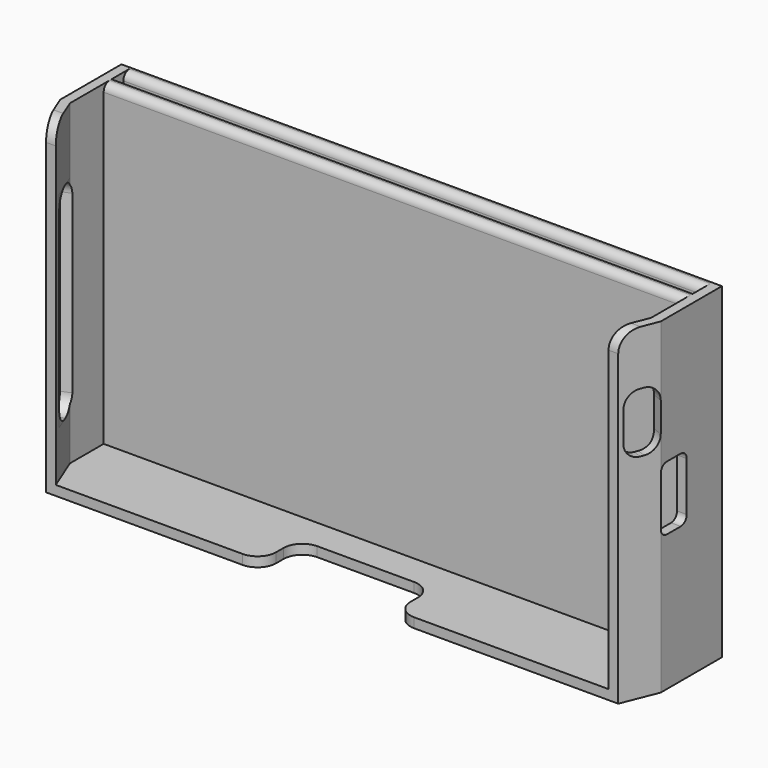
from build123d import *

# Parameters (mm, degrees)
F0_W          = 155.8
F0_H          = 85
F1_DEPTH      = 2.6
F3_DEPTH      = 85
F5_DEPTH      = 2.6
F6_W          = 8.7
F6_H          = 17.2
F7_DEPTH      = 25
F8_W          = 9
F8_H          = 16
F9_DEPTH      = 25
F10_W         = 8.5
F10_H         = 55.1
F11_DEPTH     = 25
F12_W         = 6.6
F12_H         = 87.6
F13_DEPTH     = 2.6
F14_W         = 6.6
F14_H         = 87.6
F15_DEPTH     = 2.6
F16_W         = 155.8
F16_H         = 87.6
F17_DEPTH     = 2.6
F19_W         = 36
F19_H         = 12.5
F20_DEPTH     = 25
F21_T1_DEPTH  = 2.4140393963
F21_T6_DEPTH  = 12.7075604463
F21_T12_DEPTH = 12.7075604463
F21_T18_DEPTH = 12.7075604463
F21_T24_DEPTH = 12.7075604463
F21_T30_DEPTH = 12.7075604463
F21_T36_DEPTH = 12.7075604463
F22_R         = 4
F23_T1_DEPTH  = 2.6
F23_T6_DEPTH  = 2.6
F23_T12_DEPTH = 2.6
F23_T17_DEPTH = 2.6
F23_T23_DEPTH = 2.6
F24_R         = 5
F25_R         = 2
F26_R         = 5


# Not quite as in the source:
# - a fillet or chamfer that OpenCascade refuses, or shapes differently, is made with other operations: its cross-section is extruded or revolved along the edge and cut away or added


with BuildPart() as f1:
    # F0 (on Front) → F1 (new body)
    with BuildSketch(Plane.XZ):
        Rectangle(F0_W, F0_H)
    extrude(amount=F1_DEPTH)

    # F2 (on face) → F3 (join)
    with BuildSketch(Plane.XY.offset(42.5)):
        Polygon((-77.9, -13.9), (-77.9, -2.6), (-77.9, 0), (-80.5, 0), (-80.5, -13.9), align=None)
        Polygon((-74.1, -23.4), (-77.9, -13.9), (-80.5, -13.9), (-76.7, -23.4), align=None)
        Polygon((77.9, 0), (77.9, -2.6), (77.9, -13.9), (74.1, -23.4), (76.7, -23.4), (80.5, -13.9), (80.5, 0), align=None)
    extrude(amount=-F3_DEPTH)

    # F4 (on face) → F5 (join)
    with BuildSketch(Plane(origin=(0, 0, -42.5), x_dir=(1, 0, 0), z_dir=(0, 0, -1))):
        Polygon((74.1, 23.4), (-74.1, 23.4), (-77.9, 13.9), (-77.9, 2.6), (77.9, 2.6), (77.9, 13.9), align=None)
        Polygon((-77.9, 13.9), (-74.1, 23.4), (-76.7, 23.4), (-80.5, 13.9), (-80.5, 0), (80.5, 0), (80.5, 13.9), (76.7, 23.4), (74.1, 23.4), (77.9, 13.9), (77.9, 2.6), (-77.9, 2.6), align=None)
    extrude(amount=F5_DEPTH)

    # F6 (on face) → F7 (cut)
    with BuildSketch(Plane.YZ.offset(80.5)):
        with Locations((-9.55, 0)):
            Rectangle(F6_W, F6_H)
    extrude(amount=-F7_DEPTH, mode=Mode.SUBTRACT)

    # F8 (on face) → F9 (cut)
    with BuildSketch(Plane(origin=(74.1896551724, -29.675862069, 0), x_dir=(0.3713906764, 0.9284766909, 0), z_dir=(0.9284766909, -0.3713906764, 0))):
        with Locations((12.4911234432, 19.9)):
            Rectangle(F8_W, F8_H)
    extrude(amount=-F9_DEPTH, mode=Mode.SUBTRACT)

    # F10 (on face) → F11 (cut)
    with BuildSketch(Plane(origin=(-74.1896551724, -29.675862069, 0), x_dir=(0.3713906764, -0.9284766909, 0), z_dir=(-0.9284766909, -0.3713906764, 0))):
        with Locations((-12.5093103096, -2.65)):
            Rectangle(F10_W, F10_H)
    extrude(amount=-F11_DEPTH, mode=Mode.SUBTRACT)

    # F12 (on face) → F13 (join)
    with BuildSketch(Plane(origin=(-80.5, 0, 0), x_dir=(0, -1, 0), z_dir=(-1, 0, 0))):
        with Locations((-3.3, -1.3)):
            Rectangle(F12_W, F12_H)
    extrude(amount=-F13_DEPTH)

    # F14 (on face) → F15 (join)
    with BuildSketch(Plane.YZ.offset(80.5)):
        with Locations((3.3, -1.3)):
            Rectangle(F14_W, F14_H)
    extrude(amount=-F15_DEPTH)

    # F16 (on face) → F17 (join)
    with BuildSketch(Plane(origin=(0, 6.6, 0), x_dir=(-1, 0, 0), z_dir=(0, 1, 0))):
        with Locations((0, -1.3)):
            Rectangle(F16_W, F16_H)
    extrude(amount=-F17_DEPTH)

    # F18: union 

    # F19 (on face) → F20 (cut)
    with BuildSketch(Plane(origin=(0, 0, -45.1), x_dir=(1, 0, 0), z_dir=(0, 0, -1))):
        with Locations((-1, 17.15)):
            Rectangle(F19_W, F19_H)
    extrude(amount=-F20_DEPTH, mode=Mode.SUBTRACT)

    # F21: fillet of radius 4 on 4 edges, made by hand

    # F21_s2 → F21_t1 (join)
    with BuildSketch(Plane(origin=(-74.1896551724, -29.675862069, 0), x_dir=(0, 0, 1), z_dir=(0.9284766909, 0.3713906764, 0))):
        with BuildLine():
            ThreePointArc((-30.2, -12.2593103096), (-29.0284271247, -9.4308831849), (-26.2, -8.2593103096))
            Line((-26.2, -8.2593103096), (-30.2, -8.2593103096))
            Line((-30.2, -8.2593103096), (-30.2, -12.2593103096))
        make_face()
        with BuildLine():
            ThreePointArc((24.9, -12.2593103096), (23.7284271247, -9.4308831849), (20.9, -8.2593103096))
            Line((20.9, -8.2593103096), (24.9, -8.2593103096))
            Line((24.9, -8.2593103096), (24.9, -12.2593103096))
        make_face()
    extrude(amount=F21_T1_DEPTH)


with BuildPart() as f21_tool4:
    # F21_s5 → F21_t6 (new body)
    with BuildSketch(Plane(origin=(-74.1896551724, -29.675862069, 0), x_dir=(0, 0, 1), z_dir=(0.9284766909, 0.3713906764, 0))):
        with BuildLine():
            ThreePointArc((-30.2, -12.7593103096), (-29.0284271247, -15.5877374344), (-26.2, -16.7593103096))
            Line((-26.2, -16.7593103096), (-30.2, -16.7593103096))
            Line((-30.2, -16.7593103096), (-30.2, -12.7593103096))
        make_face()
    extrude(amount=F21_T6_DEPTH)

    split(bisect_by=Plane.YZ.offset(-77.9), keep=Keep.BOTTOM)

    split(bisect_by=Plane(origin=(-71.9482758621, -28.7793103448, 0), x_dir=(0, 0, 1), z_dir=(-0.9284766909, -0.3713906764, 0)), keep=Keep.TOP)


with BuildPart() as f1_1:
    add(f1.part)

    # F21_t3: union F21_tool4
    add(f21_tool4.part)


with BuildPart() as f21_tool10:
    # F21_s11 → F21_t12 (new body)
    with BuildSketch(Plane(origin=(-74.1896551724, -29.675862069, 0), x_dir=(0, 0, 1), z_dir=(0.9284766909, 0.3713906764, 0))):
        with BuildLine():
            ThreePointArc((-30.2, -12.7593103096), (-29.0284271247, -15.5877374344), (-26.2, -16.7593103096))
            Line((-26.2, -16.7593103096), (-30.2, -16.7593103096))
            Line((-30.2, -16.7593103096), (-30.2, -12.7593103096))
        make_face()
    extrude(amount=F21_T12_DEPTH)

    split(bisect_by=Plane.YZ.offset(-77.9), keep=Keep.BOTTOM)

    split(bisect_by=Plane(origin=(-71.9482758621, -28.7793103448, 0), x_dir=(0, 0, 1), z_dir=(0.9284766909, 0.3713906764, 0)), keep=Keep.TOP)


with BuildPart() as f1_2:
    add(f1_1.part)

    # F21_t9: union F21_tool10
    add(f21_tool10.part)


with BuildPart() as f21_tool16:
    # F21_s17 → F21_t18 (new body)
    with BuildSketch(Plane(origin=(-74.1896551724, -29.675862069, 0), x_dir=(0, 0, 1), z_dir=(0.9284766909, 0.3713906764, 0))):
        with BuildLine():
            ThreePointArc((-30.2, -12.7593103096), (-29.0284271247, -15.5877374344), (-26.2, -16.7593103096))
            Line((-26.2, -16.7593103096), (-30.2, -16.7593103096))
            Line((-30.2, -16.7593103096), (-30.2, -12.7593103096))
        make_face()
    extrude(amount=F21_T18_DEPTH)

    split(bisect_by=Plane.YZ.offset(-77.9), keep=Keep.TOP)

    split(bisect_by=Plane(origin=(-71.9482758621, -28.7793103448, 0), x_dir=(0, 0, 1), z_dir=(-0.9284766909, -0.3713906764, 0)), keep=Keep.TOP)


with BuildPart() as f1_3:
    add(f1_2.part)

    # F21_t15: union F21_tool16
    add(f21_tool16.part)


with BuildPart() as f21_tool22:
    # F21_s23 → F21_t24 (new body)
    with BuildSketch(Plane(origin=(-74.1896551724, -29.675862069, 0), x_dir=(0, 0, 1), z_dir=(0.9284766909, 0.3713906764, 0))):
        with BuildLine():
            ThreePointArc((20.9, -16.7593103096), (23.7284271247, -15.5877374344), (24.9, -12.7593103096))
            Line((24.9, -12.7593103096), (24.9, -16.7593103096))
            Line((24.9, -16.7593103096), (20.9, -16.7593103096))
        make_face()
    extrude(amount=F21_T24_DEPTH)

    split(bisect_by=Plane.YZ.offset(-77.9), keep=Keep.BOTTOM)

    split(bisect_by=Plane(origin=(-71.9482758621, -28.7793103448, 0), x_dir=(0, 0, 1), z_dir=(-0.9284766909, -0.3713906764, 0)), keep=Keep.TOP)


with BuildPart() as f1_4:
    add(f1_3.part)

    # F21_t21: union F21_tool22
    add(f21_tool22.part)


with BuildPart() as f21_tool28:
    # F21_s29 → F21_t30 (new body)
    with BuildSketch(Plane(origin=(-74.1896551724, -29.675862069, 0), x_dir=(0, 0, 1), z_dir=(0.9284766909, 0.3713906764, 0))):
        with BuildLine():
            ThreePointArc((20.9, -16.7593103096), (23.7284271247, -15.5877374344), (24.9, -12.7593103096))
            Line((24.9, -12.7593103096), (24.9, -16.7593103096))
            Line((24.9, -16.7593103096), (20.9, -16.7593103096))
        make_face()
    extrude(amount=F21_T30_DEPTH)

    split(bisect_by=Plane.YZ.offset(-77.9), keep=Keep.TOP)

    split(bisect_by=Plane(origin=(-71.9482758621, -28.7793103448, 0), x_dir=(0, 0, 1), z_dir=(-0.9284766909, -0.3713906764, 0)), keep=Keep.TOP)


with BuildPart() as f1_5:
    add(f1_4.part)

    # F21_t27: union F21_tool28
    add(f21_tool28.part)


with BuildPart() as f21_tool34:
    # F21_s35 → F21_t36 (new body)
    with BuildSketch(Plane(origin=(-74.1896551724, -29.675862069, 0), x_dir=(0, 0, 1), z_dir=(0.9284766909, 0.3713906764, 0))):
        with BuildLine():
            ThreePointArc((20.9, -16.7593103096), (23.7284271247, -15.5877374344), (24.9, -12.7593103096))
            Line((24.9, -12.7593103096), (24.9, -16.7593103096))
            Line((24.9, -16.7593103096), (20.9, -16.7593103096))
        make_face()
    extrude(amount=F21_T36_DEPTH)

    split(bisect_by=Plane.YZ.offset(-77.9), keep=Keep.BOTTOM)

    split(bisect_by=Plane(origin=(-71.9482758621, -28.7793103448, 0), x_dir=(0, 0, 1), z_dir=(0.9284766909, 0.3713906764, 0)), keep=Keep.TOP)


with BuildPart() as f1_6:
    add(f1_5.part)

    # F21_t33: union F21_tool34
    add(f21_tool34.part)

    # F22 (call 1 of 4: OpenCascade refuses the feature's edges together)
    f22_edges = [f1_6.edges().sort_by_distance(p)[0] for p in [
        (76.036794, -21.808014, 11.9),
    ]]
    fillet(f22_edges, radius=F22_R)

    # F22#2 (call 2 of 4)
    f22_2_edges = [f1_6.edges().sort_by_distance(p)[0] for p in [
        (79.2, -13.38, 11.9),
    ]]
    fillet(f22_2_edges, radius=F22_R)

    # F22#3 (call 3 of 4)
    f22_3_edges = [f1_6.edges().sort_by_distance(p)[0] for p in [
        (76.036794, -21.808014, 27.9),
    ]]
    fillet(f22_3_edges, radius=F22_R)

    # F22#4 (call 4 of 4)
    f22_4_edges = [f1_6.edges().sort_by_distance(p)[0] for p in [
        (79.2, -13.38, 27.9),
    ]]
    fillet(f22_4_edges, radius=F22_R)

    # F23: fillet of radius 2 on 4 edges, made by hand

    # F23_s2 → F23_t1 (join)
    with BuildSketch(Plane.YZ.offset(77.9)):
        with BuildLine():
            ThreePointArc((-7.2, 8.6), (-5.7857864376, 8.0142135624), (-5.2, 6.6))
            Line((-5.2, 6.6), (-5.2, 8.6))
            Line((-5.2, 8.6), (-7.2, 8.6))
        make_face()
        with BuildLine():
            ThreePointArc((-5.2, -6.6), (-5.7857864376, -8.0142135624), (-7.2, -8.6))
            Line((-7.2, -8.6), (-5.2, -8.6))
            Line((-5.2, -8.6), (-5.2, -6.6))
        make_face()
    extrude(amount=F23_T1_DEPTH)


with BuildPart() as f23_tool4:
    # F23_s5 → F23_t6 (new body)
    with BuildSketch(Plane.YZ.offset(80.5)):
        with BuildLine():
            ThreePointArc((-13.9, 6.6), (-13.3142135624, 8.0142135624), (-11.9, 8.6))
            Line((-11.9, 8.6), (-13.9, 8.6))
            Line((-13.9, 8.6), (-13.9, 6.6))
        make_face()
    extrude(amount=-F23_T6_DEPTH)

    split(bisect_by=Plane(origin=(74.1896551724, -29.675862069, 0), x_dir=(0, 0, 1), z_dir=(-0.9284766909, 0.3713906764, 0)), keep=Keep.TOP)

    split(bisect_by=Plane(origin=(71.9482758621, -28.7793103448, 0), x_dir=(0, 0, 1), z_dir=(0.9284766909, -0.3713906764, 0)), keep=Keep.TOP)


with BuildPart() as f1_7:
    add(f1_6.part)

    # F23_t3: union F23_tool4
    add(f23_tool4.part)


with BuildPart() as f23_tool10:
    # F23_s11 → F23_t12 (new body)
    with BuildSketch(Plane.YZ.offset(80.5)):
        with BuildLine():
            ThreePointArc((-13.9, 6.6), (-13.3142135624, 8.0142135624), (-11.9, 8.6))
            Line((-11.9, 8.6), (-13.9, 8.6))
            Line((-13.9, 8.6), (-13.9, 6.6))
        make_face()
    extrude(amount=-F23_T12_DEPTH)

    split(bisect_by=Plane(origin=(71.9482758621, -28.7793103448, 0), x_dir=(0, 0, 1), z_dir=(-0.9284766909, 0.3713906764, 0)), keep=Keep.TOP)


with BuildPart() as f1_8:
    add(f1_7.part)

    # F23_t9: union F23_tool10
    add(f23_tool10.part)


with BuildPart() as f23_tool15:
    # F23_s16 → F23_t17 (new body)
    with BuildSketch(Plane.YZ.offset(80.5)):
        with BuildLine():
            ThreePointArc((-13.9, -6.6), (-13.3142135624, -8.0142135624), (-11.9, -8.6))
            Line((-11.9, -8.6), (-13.9, -8.6))
            Line((-13.9, -8.6), (-13.9, -6.6))
        make_face()
    extrude(amount=-F23_T17_DEPTH)

    split(bisect_by=Plane(origin=(74.1896551724, -29.675862069, 0), x_dir=(0, 0, 1), z_dir=(-0.9284766909, 0.3713906764, 0)), keep=Keep.TOP)

    split(bisect_by=Plane(origin=(71.9482758621, -28.7793103448, 0), x_dir=(0, 0, 1), z_dir=(0.9284766909, -0.3713906764, 0)), keep=Keep.TOP)


with BuildPart() as f1_9:
    add(f1_8.part)

    # F23_t14: union F23_tool15
    add(f23_tool15.part)


with BuildPart() as f23_tool21:
    # F23_s22 → F23_t23 (new body)
    with BuildSketch(Plane.YZ.offset(80.5)):
        with BuildLine():
            ThreePointArc((-13.9, -6.6), (-13.3142135624, -8.0142135624), (-11.9, -8.6))
            Line((-11.9, -8.6), (-13.9, -8.6))
            Line((-13.9, -8.6), (-13.9, -6.6))
        make_face()
    extrude(amount=-F23_T23_DEPTH)

    split(bisect_by=Plane(origin=(71.9482758621, -28.7793103448, 0), x_dir=(0, 0, 1), z_dir=(-0.9284766909, 0.3713906764, 0)), keep=Keep.TOP)


with BuildPart() as f1_10:
    add(f1_9.part)

    # F23_t20: union F23_tool21
    add(f23_tool21.part)

    # F24
    f24_edges = [f1_10.edges().sort_by_distance(p)[0] for p in [
        (17, -10.9, -43.8),
        (-19, -10.9, -43.8),
        (17, -23.4, -43.8),
        (-19, -23.4, -43.8),
    ]]
    fillet(f24_edges, radius=F24_R)

    # F25
    f25_edges = [f1_10.edges().sort_by_distance(p)[0] for p in [
        (0, -2.6, 42.5),
        (0, 4, 42.5),
    ]]
    fillet(f25_edges, radius=F25_R)

    # F26
    f26_edges = [f1_10.edges().sort_by_distance(p)[0] for p in [
        (-75.4, -23.4, 42.5),
        (75.4, -23.4, 42.5),
    ]]
    fillet(f26_edges, radius=F26_R)


solid = f1_10.part
